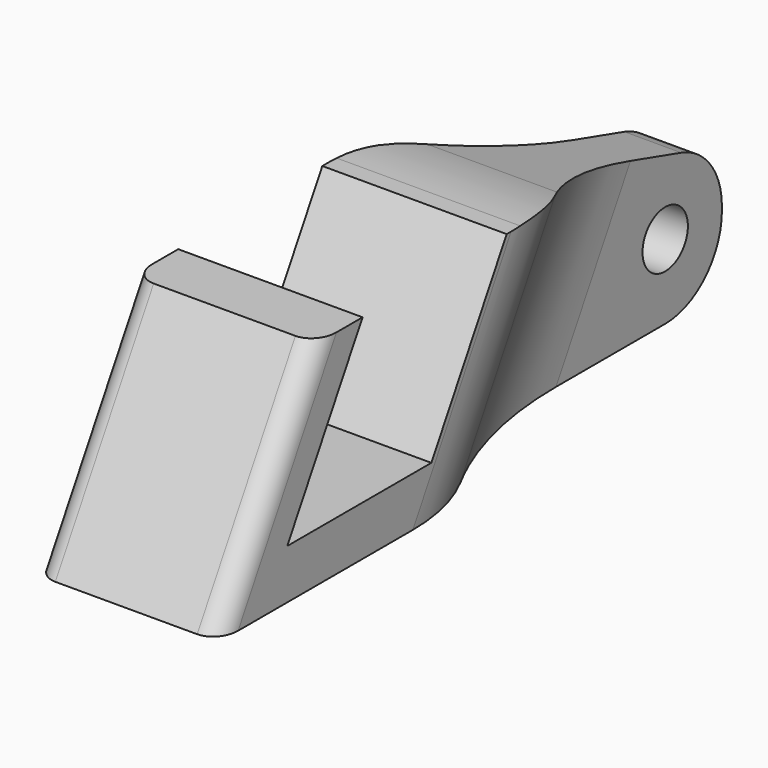
from build123d import *

# Parameters (mm, degrees)
F1_DEPTH     = 15
F3_DEPTH     = 25
F4_DEPTH     = 4.5
F6_DEPTH     = 4.5
F7_T4_DEPTH  = 80.5166313745
F7_T10_DEPTH = 80.5166313745
F8_SIZE2     = 20.5
F8_SIZE      = 6
F9_R         = 1.5
F10_R        = 10
F11_R        = 20
F12_R        = 5
F13_R        = 2
F14_DEPTH    = 25


# Not quite as in the source:
# - a fillet or chamfer that OpenCascade refuses, or shapes differently, is made with other operations: its cross-section is extruded or revolved along the edge and cut away or added


with BuildPart() as f1:
    # F0 (on Top) → F1 (new body)
    with BuildSketch(Plane.XY):
        Polygon((-6.5, 12), (-6.5, -25), (6.5, -25), (6.5, 12), (2, 12), (2, 25), (-2, 25), (-2, 12), align=None)
    extrude(amount=F1_DEPTH)

    # F2 (on face) → F3 (cut)
    with BuildSketch(Plane(origin=(-6.5, 0, 0), x_dir=(0, -1, 0), z_dir=(-1, 0, 0))):
        Polygon((6.2361162513, 3.5), (18.9378221735, 3.5), (12.2982940778, 15), (-0.4034118443, 15), align=None)
        Polygon((25, 15), (16.3397459622, 15), (25, 0), align=None)
    extrude(amount=-F3_DEPTH, mode=Mode.SUBTRACT)

    # F2 (on face) → F4 (cut)
    with BuildSketch(Plane(origin=(-6.5, 0, 0), x_dir=(0, -1, 0), z_dir=(-1, 0, 0))):
        Polygon((4.2153903092, 0), (2.194664367, 3.5), (-4.4448637287, 15), (-12, 15), (-12, 0), align=None)
    extrude(amount=-F4_DEPTH, mode=Mode.SUBTRACT)

    # F5 (on face) → F6 (cut)
    with BuildSketch(Plane.YZ.offset(6.5)):
        Polygon((12, 15), (4.4448637287, 15), (-4.2153903092, 0), (12, 0), align=None)
    extrude(amount=-F6_DEPTH, mode=Mode.SUBTRACT)

    # F7: fillet of radius 20 on 2 edges, made by hand


with BuildPart() as f7_tool2:
    # F7_s3 → F7_t4 (new body)
    with BuildSketch(Plane(origin=(0, -16.852878402, -29.190041646), x_dir=(1, 0, 0), z_dir=(0, 0.5, 0.8660254038))):
        with BuildLine():
            ThreePointArc((-6.5, -3.6506350946), (-3.1585563186, 2.2803856327), (-2, 8.9885895652))
            Line((-2, 8.9885895652), (-2, -3.6506350946))
            Line((-2, -3.6506350946), (-6.5, -3.6506350946))
        make_face()
    extrude(amount=F7_T4_DEPTH)

    split(bisect_by=Plane.XY.offset(15), keep=Keep.BOTTOM)

    split(bisect_by=Plane.XY, keep=Keep.TOP)


with BuildPart() as f1_1:
    add(f1.part)

    # F7_t1: union F7_tool2
    add(f7_tool2.part)


with BuildPart() as f7_tool8:
    # F7_s9 → F7_t10 (new body)
    with BuildSketch(Plane(origin=(0, 23.4054372853, 40.5394065514), x_dir=(1, 0, 0), z_dir=(0, -0.5, -0.8660254038))):
        with BuildLine():
            ThreePointArc((6.5, 3.6506350946), (3.1585563186, -2.2803856327), (2, -8.9885895652))
            Line((2, -8.9885895652), (2, 3.6506350946))
            Line((2, 3.6506350946), (6.5, 3.6506350946))
        make_face()
    extrude(amount=F7_T10_DEPTH)

    split(bisect_by=Plane.XY, keep=Keep.TOP)

    split(bisect_by=Plane.XY.offset(15), keep=Keep.BOTTOM)


with BuildPart() as f1_2:
    add(f1_1.part)

    # F7_t7: union F7_tool8
    add(f7_tool8.part)

    # F8
    f8_edges = [f1_2.edges().sort_by_distance(p)[0] for p in [
        (0, 25, 15),
    ]]
    f8_side = f1_2.faces().sort_by_distance((0, 25, 7.5))[0]
    chamfer(f8_edges, length=F8_SIZE, length2=F8_SIZE2, reference=f8_side)

    # F9
    f9_edges = [f1_2.edges().sort_by_distance(p)[0] for p in [
        (-6.5, -20.669873, 7.5),
        (6.5, -20.669873, 7.5),
    ]]
    fillet(f9_edges, radius=F9_R)

    # F10
    f10_edges = [f1_2.edges().sort_by_distance(p)[0] for p in [
        (-6.5, 0.114737, 7.5),
        (6.5, 0.114737, 7.5),
    ]]
    fillet(f10_edges, radius=F10_R)

    # F11
    f11_edges = [f1_2.edges().sort_by_distance(p)[0] for p in [
        (0, 4.5, 15),
    ]]
    fillet(f11_edges, radius=F11_R)

    # F12
    f12_edges = [f1_2.edges().sort_by_distance(p)[0] for p in [
        (0, 25, 9),
        (0, 25, 0),
    ]]
    fillet(f12_edges, radius=F12_R)

    # F13 (on face) → F14 (cut)
    with BuildSketch(Plane.YZ.offset(2)):
        with Locations((20, 5.2536562529)):
            Circle(F13_R)
    extrude(amount=-F14_DEPTH, mode=Mode.SUBTRACT)


solid = f1_2.part
